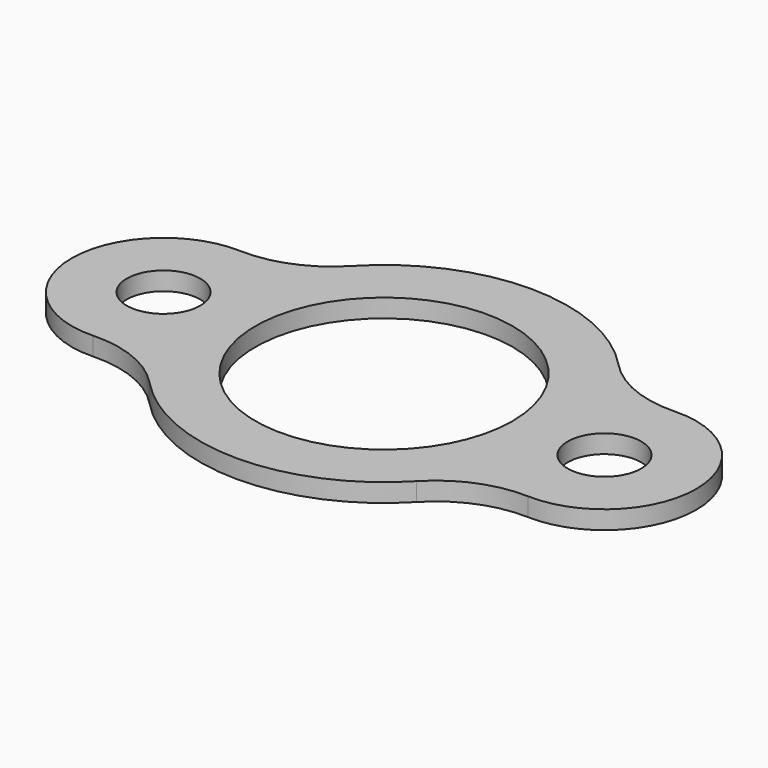
from build123d import *

# Parameters (mm, degrees)
F0_R     = 12.7
F0_R_2   = 44.45
F1_DEPTH = 6.35


# Not quite as in the source:
# - a feature names something its author has since deleted; it is built from what else it names


with BuildPart() as f1:
    # F0 (on Top) → F1 (new body)
    with BuildSketch(Plane.XY):
        with BuildLine():
            ThreePointArc((-46.13671875, 43.6308741946), (-59.3475236203, 34.5646316236), (-75.1176136364, 31.7315448688))
            ThreePointArc((-75.1176136364, 31.7315448688), (-107.95, 0), (-75.1176136364, -31.7315448688))
            ThreePointArc((-75.1176136364, -31.7315448688), (-59.3475236203, -34.5646316236), (-46.13671875, -43.6308741946))
            ThreePointArc((-46.13671875, -43.6308741946), (0, -63.5), (46.13671875, -43.6308741946))
            ThreePointArc((46.13671875, -43.6308741946), (59.3475236203, -34.5646316236), (75.1176136364, -31.7315448688))
            ThreePointArc((75.1176136364, -31.7315448688), (107.95, 0), (75.1176136364, 31.7315448688))
            ThreePointArc((75.1176136364, 31.7315448688), (59.3475236203, 34.5646316236), (46.13671875, 43.6308741946))
            ThreePointArc((46.13671875, 43.6308741946), (0, 63.5), (-46.13671875, 43.6308741946))
        make_face()
        with Locations((-76.2, 0)):
            Circle(F0_R, mode=Mode.SUBTRACT)
        Circle(F0_R_2, mode=Mode.SUBTRACT)
        with Locations((76.2, 0)):
            Circle(F0_R, mode=Mode.SUBTRACT)
    extrude(amount=F1_DEPTH)


solid = f1.part
